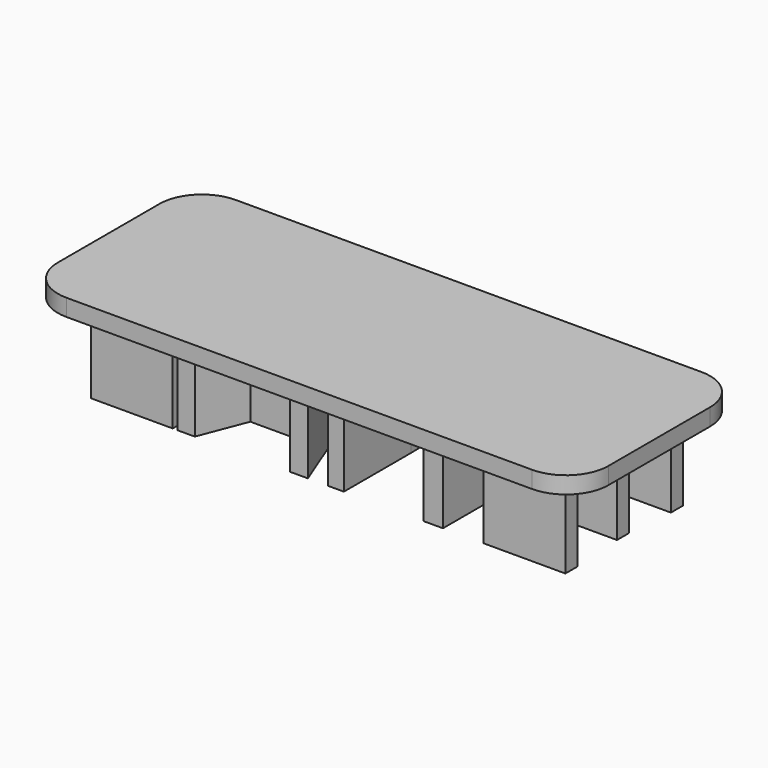
from build123d import *

# Parameters (mm, degrees)
F0_TEXT_SIZE = 30.8912396275
F1_DEPTH     = 12.7
F2_W         = 82.55
F2_H         = 31.75
F3_DEPTH     = 2.54
F4_R         = 6.35


# Not quite as in the source:
# - Text() gives the source's letters only with a copy of the font that has no kerning and outlines rounded to 1/6400 em; it was checked with that copy


with BuildPart() as f1:
    # F0 (on Top) → F1 (new body)
    with BuildSketch(Plane.XY):
        with Locations((-38.1, -11.1252)):
            Text('LANE', F0_TEXT_SIZE, font='Open Sans', text_align=(TextAlign.LEFT, TextAlign.BOTTOM))
    extrude(amount=-F1_DEPTH)


with BuildPart() as f3:
    # F2 (on Top) → F3 (new body)
    with BuildSketch(Plane.XY):
        Rectangle(F2_W, F2_H)
    extrude(amount=F3_DEPTH)

    # F4
    f4_edges = [f3.edges().sort_by_distance(p)[0] for p in [
        (-41.275, 15.875, 1.27),
        (-41.275, -15.875, 1.27),
        (41.275, -15.875, 1.27),
        (41.275, 15.875, 1.27),
    ]]
    fillet(f4_edges, radius=F4_R)


solid = Compound([f1.part, f3.part])
